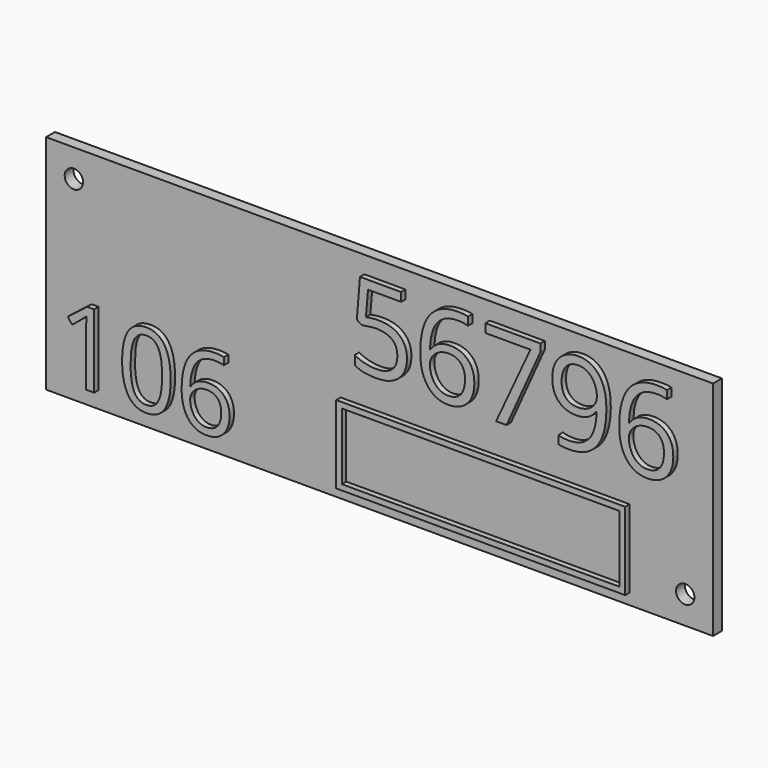
from build123d import *

# Parameters (mm, degrees)
F0_W         = 120
F0_H         = 40
F1_DEPTH     = 2
F3_D         = 3.3
F4_TEXT_SIZE = 20.871833895
F5_DEPTH     = 1
F6_TEXT_SIZE = 18.4837545126
F7_DEPTH     = 1
F8_W         = 52
F8_H         = 14
F8_W_2       = 49.99999962
F8_H_2       = 11.99999962
F9_DEPTH     = 1


# Not quite as in the source:
# - Text() gives the source's letters only with a copy of the font that has no kerning and outlines rounded to 1/6400 em; it was checked with that copy


with BuildPart() as f1:
    # F0 (on Front) → F1 (new body)
    with BuildSketch(Plane.XZ):
        Rectangle(F0_W, F0_H)
    extrude(amount=F1_DEPTH)

    # F3 (through all)
    with Locations(Plane.XZ.offset(2)):
        with Locations((-55, 15), (55, -15)):
            Hole(F3_D / 2)

    # F4 (on face) → F5 (join)
    with BuildSketch(Plane.XZ.offset(2)):
        with Locations((-5, 2)):
            Text('56796', F4_TEXT_SIZE, font='Open Sans', text_align=(TextAlign.LEFT, TextAlign.BOTTOM))
    extrude(amount=F5_DEPTH)

    # F6 (on face) → F7 (join)
    with BuildSketch(Plane.XZ.offset(2)):
        with Locations((-57, -17)):
            Text('106', F6_TEXT_SIZE, font='Open Sans', text_align=(TextAlign.LEFT, TextAlign.BOTTOM))
    extrude(amount=F7_DEPTH)

    # F8 (on face) → F9 (join)
    with BuildSketch(Plane.XZ.offset(2)):
        with Locations((19, -11)):
            Rectangle(F8_W, F8_H)
        with Locations((19, -11)):
            Rectangle(F8_W_2, F8_H_2, mode=Mode.SUBTRACT)
    extrude(amount=F9_DEPTH)


solid = f1.part
